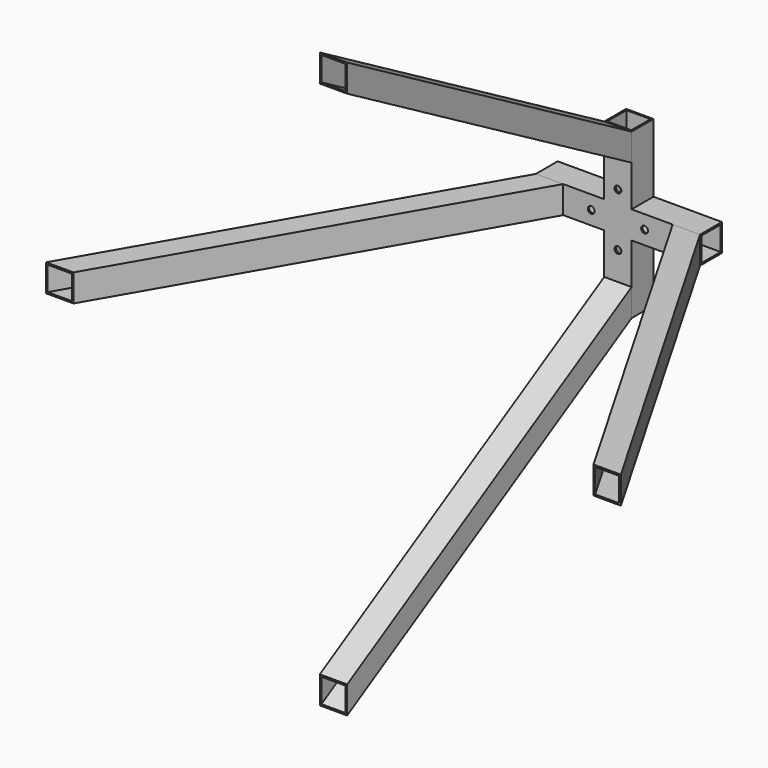
from build123d import *

# Parameters (mm, degrees)
F0_W            = 50.8
F0_H            = 50.8
F0_W_2          = 44.704
F0_H_2          = 44.704
F1_DEPTH        = 152.4
F2_W            = 50.8
F2_H            = 50.8
F2_W_2          = 44.704
F2_H_2          = 44.704
F3_DEPTH        = 127
F6_D            = 12.7
F6_COPIES_COUNT = 4
F7_W            = 50.8
F7_H            = 50.8
F7_W_2          = 44.704
F7_H_2          = 44.704
F9_COPIES_COUNT = 4


# Not quite as in the source:
# - a pattern or mirror of a feature is missing from the dataset's text; its kind, count and spacing are read off the source's solid


with BuildPart() as f1:
    # F0 (on Right) → F1 (new body, symmetric)
    with BuildSketch(Plane.YZ):
        Rectangle(F0_W, F0_H)
        Rectangle(F0_W_2, F0_H_2, mode=Mode.SUBTRACT)
    extrude(amount=F1_DEPTH, both=True)

    # F2 (on face) → F3 (join)
    with BuildSketch(Plane(origin=(0, 0, -25.4), x_dir=(1, 0, 0), z_dir=(0, 0, -1))):
        Rectangle(F2_W, F2_H)
        Rectangle(F2_W_2, F2_H_2, mode=Mode.SUBTRACT)
    extrude(amount=F3_DEPTH)

    # F4: F1 across plane


with BuildPart() as f1_1:
    add(f1.part)
    add(f1.part.mirror(Plane.XY))

    # F6 (through all)
    with Locations(Plane.XZ.offset(25.4)):
        with Locations((49.53, 0)):
            f6 = Hole(F6_D / 2)

    # F6_copies: F6 ×4 about axis
    f6_copies_axis = Axis((0, 0, 0), (0, 1, 0))
    for i in range(1, F6_COPIES_COUNT):
        add(f6.rotate(f6_copies_axis, i * 360 / F6_COPIES_COUNT), mode=Mode.SUBTRACT)


with BuildPart() as f9:
    # F9: sweep along a path in F8
    with BuildLine(Plane.XY) as f9_path:
        Line((127, -25.4), (508, -685.3113576837))
    # F7 (on face) → F9 (sweep)
    with BuildSketch(Plane.XZ.offset(25.4)):
        with Locations((127, 0)):
            Rectangle(F7_W, F7_H)
        with Locations((127, 0)):
            Rectangle(F7_W_2, F7_H_2, mode=Mode.SUBTRACT)
    sweep(path=f9_path.line)


with BuildPart() as f9_copies_1:
    # F9_copies: instance of F9
    add(f9.part.rotate(Axis((0, 0, 0), (0, 1, 0)), 1 * 360 / F9_COPIES_COUNT))


with BuildPart() as f9_copies_2:
    # F9_copies: instance of F9
    add(f9.part.rotate(Axis((0, 0, 0), (0, 1, 0)), 2 * 360 / F9_COPIES_COUNT))


with BuildPart() as f9_copies_3:
    # F9_copies: instance of F9
    add(f9.part.rotate(Axis((0, 0, 0), (0, 1, 0)), 3 * 360 / F9_COPIES_COUNT))


solid = Compound([f1_1.part, f9.part, f9_copies_1.part, f9_copies_2.part, f9_copies_3.part])
